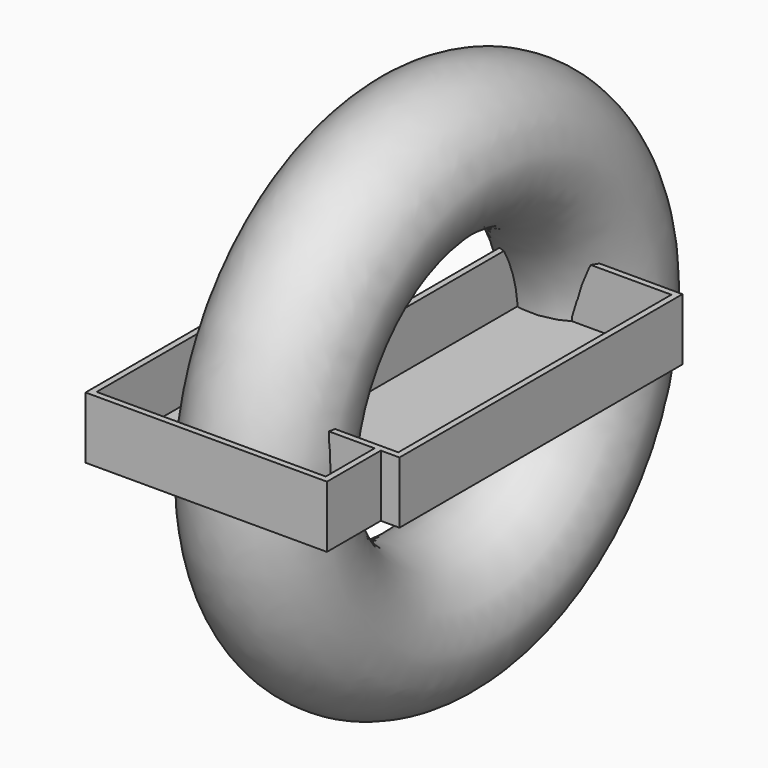
from build123d import *

# Parameters (mm, degrees)
F0_W     = 99.1622805595
F0_H     = 61.3946989179
F1_DEPTH = 25.4
F2_T     = -2.54
F3_W     = 65.9896489233
F3_H     = 145.2881251462
F4_DEPTH = 25.4
F5_T     = -2.54
F8_R     = 29.2040319406


# Not quite as in the source:
# - a shell that OpenCascade refuses in one call is made with other operations: the cavity is built on its own and cut out


with BuildPart() as f1:
    # F0 (on Top) → F1 (new body)
    with BuildSketch(Plane.XY):
        Rectangle(F0_W, F0_H)
    extrude(amount=F1_DEPTH)

    # F2
    f2_openings = [f1.faces().sort_by_distance(p)[0] for p in [
        (0, 0, 25.4),
    ]]
    offset(amount=F2_T, openings=f2_openings)

    # F3 (on Top) → F4 (join)
    with BuildSketch(Plane.XY):
        with Locations((24.260899052, 69.5941224694)):
            Rectangle(F3_W, F3_H)
    extrude(amount=F4_DEPTH)

    # F5: a shell. OpenCascade refuses it in one call, so the cavity is built on its own and cut out:
    # the body offset inwards by the wall thickness, plus a prism from it out through each open face.
    f5_core = offset(f1.part, amount=F5_T, kind=Kind.INTERSECTION, mode=Mode.PRIVATE)
    f5_exits = [f5_core.faces().sort_by_distance(p)[0] for p in [
        (24.260899, 69.594122, 22.86),
    ]]
    add(f5_core, mode=Mode.SUBTRACT)
    extrude(f5_exits, amount=-F5_T, mode=Mode.SUBTRACT)


with BuildPart() as f6_1:
    # F6: copy of F1
    add(f1.part.moved(Location((0, 65.532, 0))))


with BuildPart() as f10:
    # F10: sweep along a path in F9
    with BuildLine(Plane.YZ) as f10_path:
        CenterArc((82.7016666332, -1.5262787929), 82.715749352, 0, 360)
    # F8 (on Top) → F10 (sweep)
    with BuildSketch(Plane.XY):
        Circle(F8_R)
    sweep(path=f10_path.line)


solid = Compound([f1.part, f10.part])
